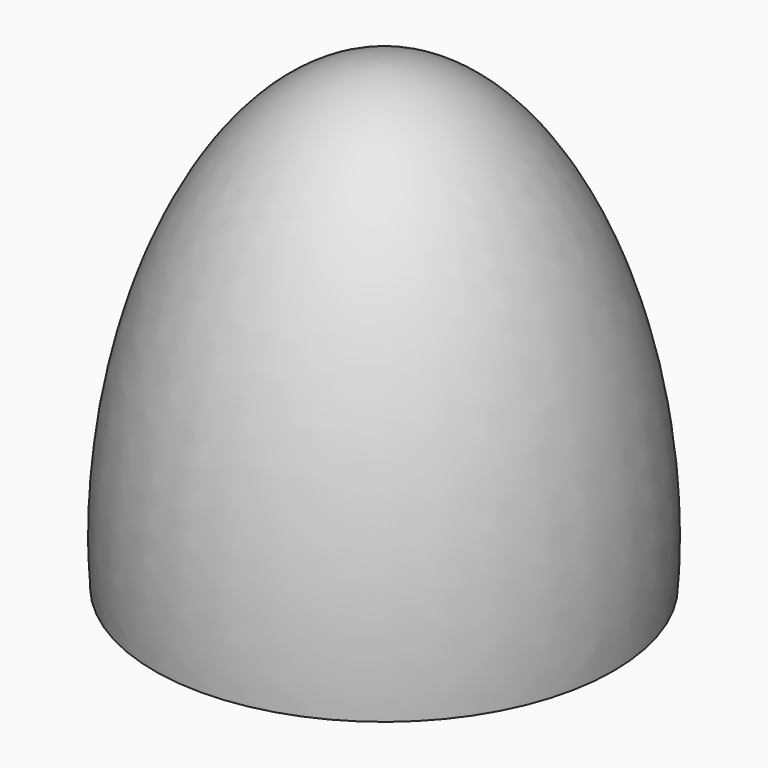
from build123d import *


# Not quite as in the source:
# - a feature names something its author has since deleted; it is built from what else it names


with BuildPart() as f2:
    # F0 (on Front) → F2 (revolve)
    with BuildSketch(Plane.XZ):
        with BuildLine():
            ThreePointArc((0, 10.5), (7.4246212025, 7.4246212025), (10.5, 0))
            Line((10.5, 0), (15, 0))
            add(Edge.make_bspline(
                [(0, 30), (9, 30), (16, 15), (15, 0)],
                knots=[0, 0, 0, 0, 33.5410196625, 33.5410196625, 33.5410196625, 33.5410196625], degree=3))
            Line((0, 30), (0, 10.5))
        make_face()
    revolve(axis=Axis((0, 0, 0), (0, 0, 1)))


solid = f2.part
